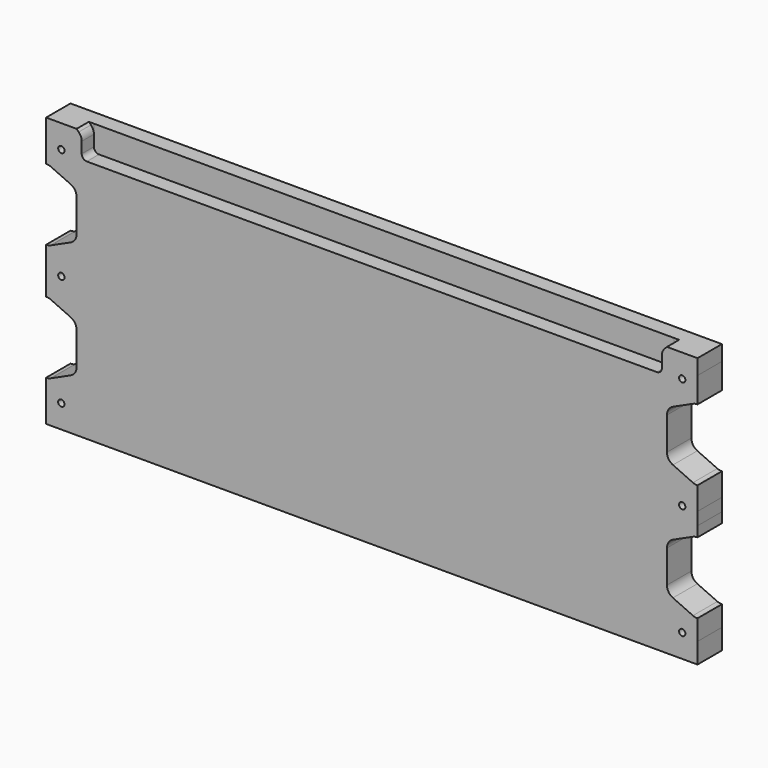
from build123d import *

# Parameters (mm, degrees)
F0_R        = 1.984375
F1_DEPTH    = 9.525
F1_FACE_R   = 1.984375
F2_DEPTH    = 9.525
F3_T1_DEPTH = 17.6900934868
F4_R        = 6.35


# Not quite as in the source:
# - a fillet or chamfer that OpenCascade refuses, or shapes differently, is made with other operations: its cross-section is extruded or revolved along the edge and cut away or added
# - ends of sketch curves that miss each other by under 0.0002 mm in the source are joined


with BuildPart() as f1:
    # F0 (on Front) → F1 (new body)
    with BuildSketch(Plane.XZ):
        with BuildLine():
            Line((192.4844258, 36.003738), (200.0250254, 36.003738))
            Line((200.0250254, 36.003738), (200.0250254, 47.116238))
            Line((200.0250254, 47.116238), (200.0250254, 50.291238))
            Line((200.0250254, 50.291238), (199.8129496538, 50.291238))
            ThreePointArc((199.8129496538, 50.291238), (198.4686550901, 50.4351625794), (197.1852981737, 50.8604121335))
            Line((197.1852981737, 50.8604121335), (184.6973485199, 56.5367601413))
            ThreePointArc((184.6973485199, 56.5367601413), (181.9860821837, 58.8797877952), (180.975, 62.3175860078))
            Line((180.975, 62.3175860078), (180.975, 82.7148899922))
            ThreePointArc((180.975, 82.7148899922), (181.9860821837, 86.1526882048), (184.6973485199, 88.4957158587))
            Line((184.6973485199, 88.4957158587), (197.1852981737, 94.1720638665))
            ThreePointArc((197.1852981737, 94.1720638665), (198.4686550901, 94.5973134206), (199.8129496538, 94.741238))
            Line((199.8129496538, 94.741238), (200.025, 94.741238))
            Line((200.025, 94.741238), (200.0250254, 110.616238))
            Line((200.0250254, 110.616238), (200.0250254, 120.141238))
            Line((200.0250254, 120.141238), (177.8000254, 120.141238))
            Line((177.8000254, 120.141238), (177.8000254, 107.441238))
            ThreePointArc((177.8000254, 107.441238), (176.8700894303, 105.1961739697), (174.6250254, 104.266238))
            Line((174.6250254, 104.266238), (-180.9749746, 104.266238))
            ThreePointArc((-180.9749746, 104.266238), (-183.2200386303, 105.1961739697), (-184.1499746, 107.441238))
            Line((-184.1499746, 107.441238), (-184.1499746, 120.141238))
            Line((-184.1499746, 120.141238), (-206.3749746, 120.141238))
            Line((-206.3749746, 120.141238), (-206.3749746, 94.741238))
            Line((-206.3749746, 94.741238), (-206.1629496538, 94.741238))
            ThreePointArc((-206.1629496538, 94.741238), (-204.8186550901, 94.5973134206), (-203.5352981737, 94.1720638665))
            Line((-203.5352981737, 94.1720638665), (-191.0473485199, 88.4957158587))
            ThreePointArc((-191.0473485199, 88.4957158587), (-188.3360821837, 86.1526882048), (-187.325, 82.7148899922))
            Line((-187.325, 82.7148899922), (-187.325, 62.3175860078))
            ThreePointArc((-187.325, 62.3175860078), (-188.3360821837, 58.8797877952), (-191.0473485199, 56.5367601413))
            Line((-191.0473485199, 56.5367601413), (-203.5352981737, 50.8604121335))
            ThreePointArc((-203.5352981737, 50.8604121335), (-204.8186550901, 50.4351625794), (-206.1629496538, 50.291238))
            Line((-206.1629496538, 50.291238), (-206.375, 50.291238))
            Line((-206.375, 50.291238), (-206.3749746, 36.003738))
            Line((-206.3749746, 36.003738), (-198.834375, 36.003738))
            ThreePointArc((-198.834375, 36.003738), (-196.85, 37.988113), (-194.865625, 36.003738))
            Line((-194.865625, 36.003738), (188.5156758, 36.003738))
            ThreePointArc((188.5156758, 36.003738), (190.5000508, 37.988113), (192.4844258, 36.003738))
        make_face()
        with Locations((-196.8500060797, 105.6372644242)):
            Circle(F0_R, mode=Mode.SUBTRACT)
        with Locations((190.5000060797, 105.6372644242)):
            Circle(F0_R, mode=Mode.SUBTRACT)
        with BuildLine():
            Line((200.025, 21.716238), (200.025, 28.066238))
            Line((200.025, 28.066238), (200.0250254, 36.003738))
            Line((200.0250254, 36.003738), (192.4844258, 36.003738))
            ThreePointArc((192.4844258, 36.003738), (190.5000508, 34.019363), (188.5156758, 36.003738))
            Line((188.5156758, 36.003738), (-194.865625, 36.003738))
            ThreePointArc((-194.865625, 36.003738), (-196.85, 34.019363), (-198.834375, 36.003738))
            Line((-198.834375, 36.003738), (-206.3749746, 36.003738))
            Line((-206.3749746, 36.003738), (-206.3749746, 21.716238))
            Line((-206.3749746, 21.716238), (-206.1629496538, 21.716238))
            ThreePointArc((-206.1629496538, 21.716238), (-204.8186550901, 21.5723134206), (-203.5352981737, 21.1470638665))
            Line((-203.5352981737, 21.1470638665), (-191.0473485199, 15.4707158587))
            ThreePointArc((-191.0473485199, 15.4707158587), (-188.3360821837, 13.1276882048), (-187.325, 9.6898899922))
            Line((-187.325, 9.6898899922), (-187.325, -10.7074139922))
            ThreePointArc((-187.325, -10.7074139922), (-188.3360821837, -14.1452122048), (-191.0473485199, -16.4882398587))
            Line((-191.0473485199, -16.4882398587), (-203.5352981737, -22.1645878665))
            ThreePointArc((-203.5352981737, -22.1645878665), (-204.8186550901, -22.5898374206), (-206.1629496538, -22.733762))
            Line((-206.1629496538, -22.733762), (-206.375, -22.733762))
            Line((-206.375, -22.733762), (-206.3749746, -48.133762))
            Line((-206.3749746, -48.133762), (200.0250254, -48.133762))
            Line((200.0250254, -48.133762), (200.0250254, -35.433762))
            Line((200.0250254, -35.433762), (200.025, -22.733762))
            Line((200.025, -22.733762), (199.8129496538, -22.733762))
            ThreePointArc((199.8129496538, -22.733762), (198.4686550901, -22.5898374206), (197.1852981737, -22.1645878665))
            Line((197.1852981737, -22.1645878665), (184.6973485199, -16.4882398587))
            ThreePointArc((184.6973485199, -16.4882398587), (181.9860821837, -14.1452122048), (180.975, -10.7074139922))
            Line((180.975, -10.7074139922), (180.975, 9.6898899922))
            ThreePointArc((180.975, 9.6898899922), (181.9860821837, 13.1276882048), (184.6973485199, 15.4707158587))
            Line((184.6973485199, 15.4707158587), (197.1852981737, 21.1470638665))
            ThreePointArc((197.1852981737, 21.1470638665), (198.4686550901, 21.5723134206), (199.8129496538, 21.716238))
            Line((199.8129496538, 21.716238), (200.025, 21.716238))
        make_face()
        with Locations((-196.8500060797, -33.6297884242)):
            Circle(F0_R, mode=Mode.SUBTRACT)
        with Locations((190.5000060797, -33.6297884242)):
            Circle(F0_R, mode=Mode.SUBTRACT)
    extrude(amount=F1_DEPTH)

    # F0 (on Front) + F1_face (on face) → F2 (join)
    with BuildSketch(Plane.XZ):
        with BuildLine():
            Line((200.025, 21.716238), (200.025, 28.066238))
            Line((200.025, 28.066238), (200.0250254, 36.003738))
            Line((200.0250254, 36.003738), (192.4844258, 36.003738))
            ThreePointArc((192.4844258, 36.003738), (190.5000508, 34.019363), (188.5156758, 36.003738))
            Line((188.5156758, 36.003738), (-194.865625, 36.003738))
            ThreePointArc((-194.865625, 36.003738), (-196.85, 34.019363), (-198.834375, 36.003738))
            Line((-198.834375, 36.003738), (-206.3749746, 36.003738))
            Line((-206.3749746, 36.003738), (-206.3749746, 21.716238))
            Line((-206.3749746, 21.716238), (-206.1629496538, 21.716238))
            ThreePointArc((-206.1629496538, 21.716238), (-204.8186550901, 21.5723134206), (-203.5352981737, 21.1470638665))
            Line((-203.5352981737, 21.1470638665), (-191.0473485199, 15.4707158587))
            ThreePointArc((-191.0473485199, 15.4707158587), (-188.3360821837, 13.1276882048), (-187.325, 9.6898899922))
            Line((-187.325, 9.6898899922), (-187.325, -10.7074139922))
            ThreePointArc((-187.325, -10.7074139922), (-188.3360821837, -14.1452122048), (-191.0473485199, -16.4882398587))
            Line((-191.0473485199, -16.4882398587), (-203.5352981737, -22.1645878665))
            ThreePointArc((-203.5352981737, -22.1645878665), (-204.8186550901, -22.5898374206), (-206.1629496538, -22.733762))
            Line((-206.1629496538, -22.733762), (-206.375, -22.733762))
            Line((-206.375, -22.733762), (-206.3749746, -48.133762))
            Line((-206.3749746, -48.133762), (200.0250254, -48.133762))
            Line((200.0250254, -48.133762), (200.0250254, -35.433762))
            Line((200.0250254, -35.433762), (200.025, -22.733762))
            Line((200.025, -22.733762), (199.8129496538, -22.733762))
            ThreePointArc((199.8129496538, -22.733762), (198.4686550901, -22.5898374206), (197.1852981737, -22.1645878665))
            Line((197.1852981737, -22.1645878665), (184.6973485199, -16.4882398587))
            ThreePointArc((184.6973485199, -16.4882398587), (181.9860821837, -14.1452122048), (180.975, -10.7074139922))
            Line((180.975, -10.7074139922), (180.975, 9.6898899922))
            ThreePointArc((180.975, 9.6898899922), (181.9860821837, 13.1276882048), (184.6973485199, 15.4707158587))
            Line((184.6973485199, 15.4707158587), (197.1852981737, 21.1470638665))
            ThreePointArc((197.1852981737, 21.1470638665), (198.4686550901, 21.5723134206), (199.8129496538, 21.716238))
            Line((199.8129496538, 21.716238), (200.025, 21.716238))
        make_face()
        with Locations((-196.8500060797, -33.6297884242)):
            Circle(F0_R, mode=Mode.SUBTRACT)
        with Locations((190.5000060797, -33.6297884242)):
            Circle(F0_R, mode=Mode.SUBTRACT)
        with BuildLine():
            Line((192.4844258, 36.003738), (200.0250254, 36.003738))
            Line((200.0250254, 36.003738), (200.0250254, 47.116238))
            Line((200.0250254, 47.116238), (200.0250254, 50.291238))
            Line((200.0250254, 50.291238), (199.8129496538, 50.291238))
            ThreePointArc((199.8129496538, 50.291238), (198.4686550901, 50.4351625794), (197.1852981737, 50.8604121335))
            Line((197.1852981737, 50.8604121335), (184.6973485199, 56.5367601413))
            ThreePointArc((184.6973485199, 56.5367601413), (181.9860821837, 58.8797877952), (180.975, 62.3175860078))
            Line((180.975, 62.3175860078), (180.975, 82.7148899922))
            ThreePointArc((180.975, 82.7148899922), (181.9860821837, 86.1526882048), (184.6973485199, 88.4957158587))
            Line((184.6973485199, 88.4957158587), (197.1852981737, 94.1720638665))
            ThreePointArc((197.1852981737, 94.1720638665), (198.4686550901, 94.5973134206), (199.8129496538, 94.741238))
            Line((199.8129496538, 94.741238), (200.025, 94.741238))
            Line((200.025, 94.741238), (200.0250254, 110.616238))
            Line((200.0250254, 110.616238), (200.0250254, 120.141238))
            Line((200.0250254, 120.141238), (177.8000254, 120.141238))
            Line((177.8000254, 120.141238), (177.8000254, 107.441238))
            ThreePointArc((177.8000254, 107.441238), (176.8700894303, 105.1961739697), (174.6250254, 104.266238))
            Line((174.6250254, 104.266238), (-180.9749746, 104.266238))
            ThreePointArc((-180.9749746, 104.266238), (-183.2200386303, 105.1961739697), (-184.1499746, 107.441238))
            Line((-184.1499746, 107.441238), (-184.1499746, 120.141238))
            Line((-184.1499746, 120.141238), (-206.3749746, 120.141238))
            Line((-206.3749746, 120.141238), (-206.3749746, 94.741238))
            Line((-206.3749746, 94.741238), (-206.1629496538, 94.741238))
            ThreePointArc((-206.1629496538, 94.741238), (-204.8186550901, 94.5973134206), (-203.5352981737, 94.1720638665))
            Line((-203.5352981737, 94.1720638665), (-191.0473485199, 88.4957158587))
            ThreePointArc((-191.0473485199, 88.4957158587), (-188.3360821837, 86.1526882048), (-187.325, 82.7148899922))
            Line((-187.325, 82.7148899922), (-187.325, 62.3175860078))
            ThreePointArc((-187.325, 62.3175860078), (-188.3360821837, 58.8797877952), (-191.0473485199, 56.5367601413))
            Line((-191.0473485199, 56.5367601413), (-203.5352981737, 50.8604121335))
            ThreePointArc((-203.5352981737, 50.8604121335), (-204.8186550901, 50.4351625794), (-206.1629496538, 50.291238))
            Line((-206.1629496538, 50.291238), (-206.375, 50.291238))
            Line((-206.375, 50.291238), (-206.3749746, 36.003738))
            Line((-206.3749746, 36.003738), (-198.834375, 36.003738))
            ThreePointArc((-198.834375, 36.003738), (-196.85, 37.988113), (-194.865625, 36.003738))
            Line((-194.865625, 36.003738), (188.5156758, 36.003738))
            ThreePointArc((188.5156758, 36.003738), (190.5000508, 37.988113), (192.4844258, 36.003738))
        make_face()
        with Locations((-196.8500060797, 105.6372644242)):
            Circle(F0_R, mode=Mode.SUBTRACT)
        with Locations((190.5000060797, 105.6372644242)):
            Circle(F0_R, mode=Mode.SUBTRACT)
        with BuildLine():
            Line((177.8000254, 107.441238), (177.8000254, 120.141238))
            Line((177.8000254, 120.141238), (-184.1499746, 120.141238))
            Line((-184.1499746, 120.141238), (-184.1499746, 107.441238))
            ThreePointArc((-184.1499746, 107.441238), (-183.2200386303, 105.1961739697), (-180.9749746, 104.266238))
            Line((-180.9749746, 104.266238), (174.6250254, 104.266238))
            ThreePointArc((174.6250254, 104.266238), (176.8700894303, 105.1961739697), (177.8000254, 107.441238))
        make_face()
    with BuildSketch(Plane(origin=(-3.1749925795, -9.525, 28.6823887968), x_dir=(1, 0, 0), z_dir=(0, -1, 0))):
        with BuildLine():
            Line((-203.2000074205, 21.6088492032), (-203.1999820205, 7.3213492032))
            Line((-203.1999820205, 7.3213492032), (-203.1999820205, -6.9661507968))
            Line((-203.1999820205, -6.9661507968), (-202.9879570743, -6.9661507968))
            ThreePointArc((-202.9879570743, -6.9661507968), (-201.6436625106, -7.1100753762), (-200.3603055942, -7.5353249303))
            Line((-200.3603055942, -7.5353249303), (-187.8723559404, -13.2116729381))
            ThreePointArc((-187.8723559404, -13.2116729381), (-185.1610896042, -15.5547005921), (-184.1500074205, -18.9924988047))
            Line((-184.1500074205, -18.9924988047), (-184.1500074205, -39.389802789))
            ThreePointArc((-184.1500074205, -39.389802789), (-185.1610896042, -42.8276010016), (-187.8723559404, -45.1706286555))
            Line((-187.8723559404, -45.1706286555), (-200.3603055942, -50.8469766634))
            ThreePointArc((-200.3603055942, -50.8469766634), (-201.6436625106, -51.2722262174), (-202.9879570743, -51.4161507968))
            Line((-202.9879570743, -51.4161507968), (-203.2000074205, -51.4161507968))
            Line((-203.2000074205, -51.4161507968), (-203.1999820205, -76.8161507968))
            Line((-203.1999820205, -76.8161507968), (203.2000179795, -76.8161507968))
            Line((203.2000179795, -76.8161507968), (203.2000179795, -64.1161507968))
            Line((203.2000179795, -64.1161507968), (203.1999925795, -51.4161507968))
            Line((203.1999925795, -51.4161507968), (202.9879422333, -51.4161507968))
            ThreePointArc((202.9879422333, -51.4161507968), (201.6436476697, -51.2722262174), (200.3602907532, -50.8469766634))
            Line((200.3602907532, -50.8469766634), (187.8723410994, -45.1706286555))
            ThreePointArc((187.8723410994, -45.1706286555), (185.1610747632, -42.8276010016), (184.1499925795, -39.389802789))
            Line((184.1499925795, -39.389802789), (184.1499925795, -18.9924988047))
            ThreePointArc((184.1499925795, -18.9924988047), (185.1610747632, -15.5547005921), (187.8723410994, -13.2116729381))
            Line((187.8723410994, -13.2116729381), (200.3602907532, -7.5353249303))
            ThreePointArc((200.3602907532, -7.5353249303), (201.6436476697, -7.1100753762), (202.9879422333, -6.9661507968))
            Line((202.9879422333, -6.9661507968), (203.1999925795, -6.9661507968))
            Line((203.1999925795, -6.9661507968), (203.1999925795, -0.6161507968))
            Line((203.1999925795, -0.6161507968), (203.2000179795, 7.3213492032))
            Line((203.2000179795, 7.3213492032), (203.2000179795, 21.6088492032))
            Line((203.2000179795, 21.6088492032), (202.9879422333, 21.6088492032))
            ThreePointArc((202.9879422333, 21.6088492032), (201.6436476697, 21.7527737826), (200.3602907532, 22.1780233366))
            Line((200.3602907532, 22.1780233366), (187.8723410994, 27.8543713445))
            ThreePointArc((187.8723410994, 27.8543713445), (185.1610747632, 30.1973989984), (184.1499925795, 33.635197211))
            Line((184.1499925795, 33.635197211), (184.1499925795, 54.0325011953))
            ThreePointArc((184.1499925795, 54.0325011953), (185.1610747632, 57.4702994079), (187.8723410994, 59.8133270619))
            Line((187.8723410994, 59.8133270619), (200.3602907532, 65.4896750697))
            ThreePointArc((200.3602907532, 65.4896750697), (201.6436476697, 65.9149246238), (202.9879422333, 66.0588492032))
            Line((202.9879422333, 66.0588492032), (203.1999925795, 66.0588492032))
            Line((203.1999925795, 66.0588492032), (203.2000179795, 81.9338492032))
            Line((203.2000179795, 81.9338492032), (203.2000179795, 91.4588492032))
            Line((203.2000179795, 91.4588492032), (180.9750179795, 91.4588492032))
            Line((180.9750179795, 91.4588492032), (180.9750179795, 78.7588492032))
            ThreePointArc((180.9750179795, 78.7588492032), (180.0450820098, 76.5137851729), (177.8000179795, 75.5838492032))
            Line((177.8000179795, 75.5838492032), (-177.7999820205, 75.5838492032))
            ThreePointArc((-177.7999820205, 75.5838492032), (-180.0450460508, 76.5137851729), (-180.9749820205, 78.7588492032))
            Line((-180.9749820205, 78.7588492032), (-180.9749820205, 91.4588492032))
            Line((-180.9749820205, 91.4588492032), (-203.1999820205, 91.4588492032))
            Line((-203.1999820205, 91.4588492032), (-203.1999820205, 66.0588492032))
            Line((-203.1999820205, 66.0588492032), (-202.9879570743, 66.0588492032))
            ThreePointArc((-202.9879570743, 66.0588492032), (-201.6436625106, 65.9149246238), (-200.3603055942, 65.4896750697))
            Line((-200.3603055942, 65.4896750697), (-187.8723559404, 59.8133270619))
            ThreePointArc((-187.8723559404, 59.8133270619), (-185.1610896042, 57.4702994079), (-184.1500074205, 54.0325011953))
            Line((-184.1500074205, 54.0325011953), (-184.1500074205, 33.635197211))
            ThreePointArc((-184.1500074205, 33.635197211), (-185.1610896042, 30.1973989984), (-187.8723559404, 27.8543713445))
            Line((-187.8723559404, 27.8543713445), (-200.3603055942, 22.1780233366))
            ThreePointArc((-200.3603055942, 22.1780233366), (-201.6436625106, 21.7527737826), (-202.9879570743, 21.6088492032))
            Line((-202.9879570743, 21.6088492032), (-203.2000074205, 21.6088492032))
        make_face()
        with Locations((-193.6750074205, 7.3213492032)):
            Circle(F1_FACE_R, mode=Mode.SUBTRACT)
        with Locations((193.6750433795, 7.3213492032)):
            Circle(F1_FACE_R, mode=Mode.SUBTRACT)
        with Locations((-193.6750135002, 76.9548756274)):
            Circle(F1_FACE_R, mode=Mode.SUBTRACT)
        with Locations((193.6749986592, 76.9548756274)):
            Circle(F1_FACE_R, mode=Mode.SUBTRACT)
        with Locations((193.6749986592, -62.312177221)):
            Circle(F1_FACE_R, mode=Mode.SUBTRACT)
        with Locations((-193.6750135002, -62.312177221)):
            Circle(F1_FACE_R, mode=Mode.SUBTRACT)
    extrude(amount=-F2_DEPTH)

    # F3: chamfer of 3.175 on 2 edges, made by hand

    # F3_s2 → F3_t1 (cut)
    with BuildSketch(Plane.XZ):
        Polygon((-184.1499746, 116.966238), (-187.3249746, 120.141238), (-184.1499746, 120.141238), align=None)
        Polygon((180.9750254, 120.141238), (177.8000254, 116.966238), (177.8000254, 120.141238), align=None)
    extrude(amount=F3_T1_DEPTH, mode=Mode.SUBTRACT)

    # F4
    f4_edges = [f1.edges().sort_by_distance(p)[0] for p in [
        (-184.149975, -4.7625, 116.966238),
        (177.800025, -4.7625, 116.966238),
    ]]
    fillet(f4_edges, radius=F4_R)


solid = f1.part
